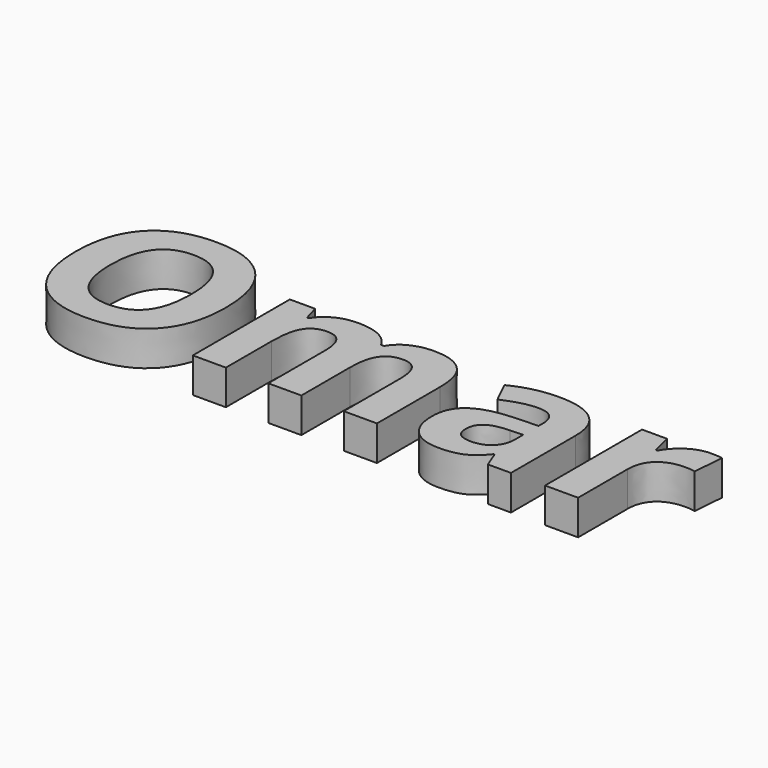
from build123d import *

# Parameters (mm, degrees)
F0_TEXT_SIZE = 161.6628012723
F1_DEPTH     = 25.4


# Not quite as in the source:
# - Text() gives the source's letters only with a copy of the font that has no kerning and outlines rounded to 1/6400 em; it was checked with that copy


with BuildPart() as f1:
    # F0 (on Top) → F1 (new body)
    with BuildSketch(Plane.XY):
        with Locations((-192.225381732, -38.4979061782)):
            Text('Omar', F0_TEXT_SIZE, font='Open Sans', font_style=FontStyle.BOLD, text_align=(TextAlign.LEFT, TextAlign.BOTTOM))
    extrude(amount=F1_DEPTH)


solid = f1.part
